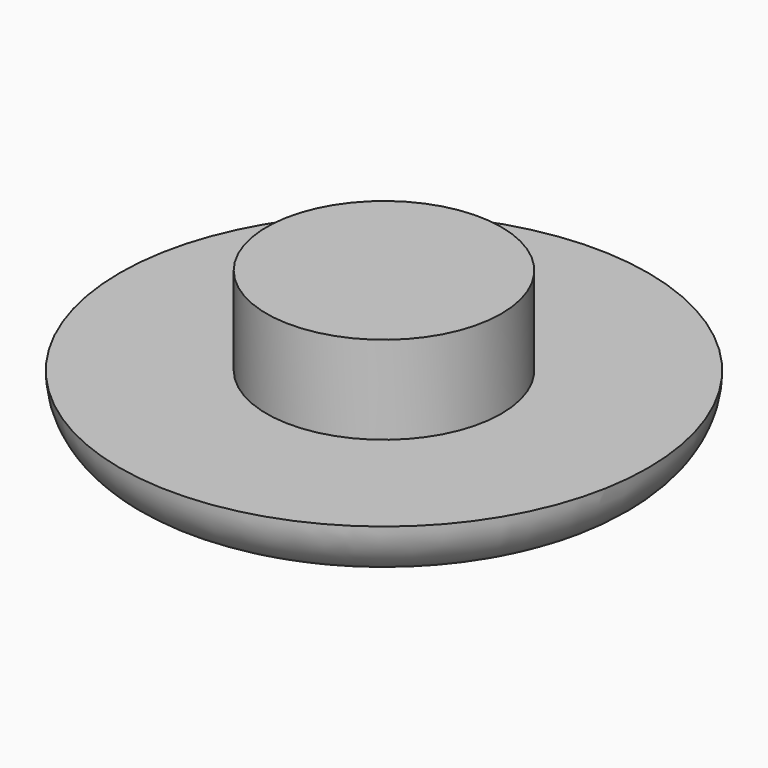
from build123d import *

# Parameters (mm, degrees)
F0_R         = 9
F1_DEPTH     = 2
F2_R         = 4
F3_DEPTH     = 3
F4_R         = 1.99999
F5_TEXT_SIZE = 13.162180731
F6_DEPTH     = 1


# Not quite as in the source:
# - a fillet or chamfer is up to 0.001 mm smaller than in the source, because OpenCascade refuses the exact size
# - Text() gives the source's letters only with a copy of the font that has no kerning and outlines rounded to 1/6400 em; it was checked with that copy


with BuildPart() as f1:
    # F0 (on Top) → F1 (new body)
    with BuildSketch(Plane.XY):
        Circle(F0_R)
    extrude(amount=F1_DEPTH)

    # F2 (on face) → F3 (join)
    with BuildSketch(Plane.XY.offset(2)):
        Circle(F2_R)
    extrude(amount=F3_DEPTH)

    # F4 (radius 2 in the source; OpenCascade refuses exactly that, so slightly less here)
    f4_edges = [f1.edges().sort_by_distance(p)[0] for p in [
        (-9, 0, 0),
    ]]
    fillet(f4_edges, radius=F4_R)

    # F5 (on face) → F6 (cut)
    with BuildSketch(Plane(origin=(0, 0, 0), x_dir=(1, 0, 0), z_dir=(0, 0, -1))):
        with Locations((-5.2407336364, -4.8362194098)):
            Text('O', F5_TEXT_SIZE, font='Open Sans', text_align=(TextAlign.LEFT, TextAlign.BOTTOM))
    extrude(amount=-F6_DEPTH, mode=Mode.SUBTRACT)


solid = f1.part
